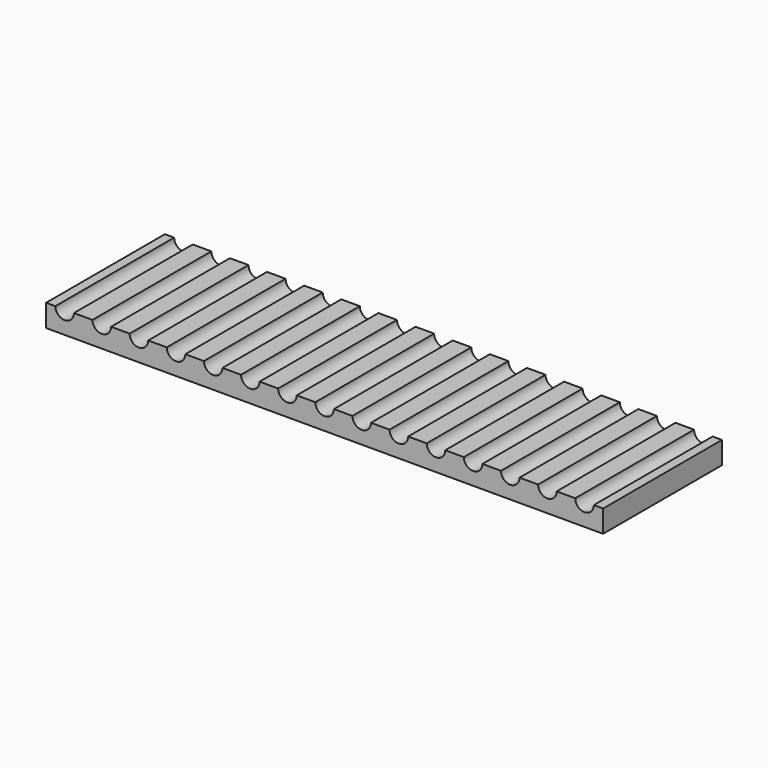
from build123d import *

# Parameters (mm, degrees)
F0_W     = 150
F0_H     = 6
F1_DEPTH = 40
F3_DEPTH = 40.001


with BuildPart() as f1:
    # F0 (on Front) → F1 (new body)
    with BuildSketch(Plane.XZ):
        with Locations((75, 3)):
            Rectangle(F0_W, F0_H)
    extrude(amount=-F1_DEPTH)

    # F2 (on face) → F3 (cut, through all)
    with BuildSketch(Plane.XZ):
        with BuildLine():
            ThreePointArc((2.5, 6), (5, 3.5), (7.5, 6))
            Line((7.5, 6), (2.5, 6))
        make_face()
        with BuildLine():
            Line((17.5, 6), (12.5, 6))
            ThreePointArc((12.5, 6), (15, 3.5), (17.5, 6))
        make_face()
        with BuildLine():
            Line((27.5, 6), (22.5, 6))
            ThreePointArc((22.5, 6), (25, 3.5), (27.5, 6))
        make_face()
        with BuildLine():
            Line((37.5, 6), (32.5, 6))
            ThreePointArc((32.5, 6), (35, 3.5), (37.5, 6))
        make_face()
        with BuildLine():
            Line((142.5, 6), (147.5, 6))
            ThreePointArc((147.5, 6), (145, 8.5), (142.5, 6))
        make_face()
        with BuildLine():
            ThreePointArc((142.5, 6), (145, 3.5), (147.5, 6))
            Line((147.5, 6), (142.5, 6))
        make_face()
        with BuildLine():
            Line((47.5, 6), (42.5, 6))
            ThreePointArc((42.5, 6), (45, 3.5), (47.5, 6))
        make_face()
        with BuildLine():
            Line((132.5, 6), (137.5, 6))
            ThreePointArc((137.5, 6), (135, 8.5), (132.5, 6))
        make_face()
        with BuildLine():
            ThreePointArc((132.5, 6), (135, 3.5), (137.5, 6))
            Line((137.5, 6), (132.5, 6))
        make_face()
        with BuildLine():
            Line((57.5, 6), (52.5, 6))
            ThreePointArc((52.5, 6), (55, 3.5), (57.5, 6))
        make_face()
        with BuildLine():
            Line((122.5, 6), (127.5, 6))
            ThreePointArc((127.5, 6), (125, 8.5), (122.5, 6))
        make_face()
        with BuildLine():
            ThreePointArc((122.5, 6), (125, 3.5), (127.5, 6))
            Line((127.5, 6), (122.5, 6))
        make_face()
        with BuildLine():
            Line((67.5, 6), (62.5, 6))
            ThreePointArc((62.5, 6), (65, 3.5), (67.5, 6))
        make_face()
        with BuildLine():
            Line((112.5, 6), (117.5, 6))
            ThreePointArc((117.5, 6), (115, 8.5), (112.5, 6))
        make_face()
        with BuildLine():
            ThreePointArc((112.5, 6), (115, 3.5), (117.5, 6))
            Line((117.5, 6), (112.5, 6))
        make_face()
        with BuildLine():
            Line((77.5, 6), (72.5, 6))
            ThreePointArc((72.5, 6), (75, 3.5), (77.5, 6))
        make_face()
        with BuildLine():
            ThreePointArc((102.5, 6), (105, 3.5), (107.5, 6))
            Line((107.5, 6), (102.5, 6))
        make_face()
        with BuildLine():
            Line((87.5, 6), (82.5, 6))
            ThreePointArc((82.5, 6), (85, 3.5), (87.5, 6))
        make_face()
        with BuildLine():
            ThreePointArc((92.5, 6), (95, 3.5), (97.5, 6))
            Line((97.5, 6), (92.5, 6))
        make_face()
    extrude(amount=-F3_DEPTH, mode=Mode.SUBTRACT)


solid = f1.part
